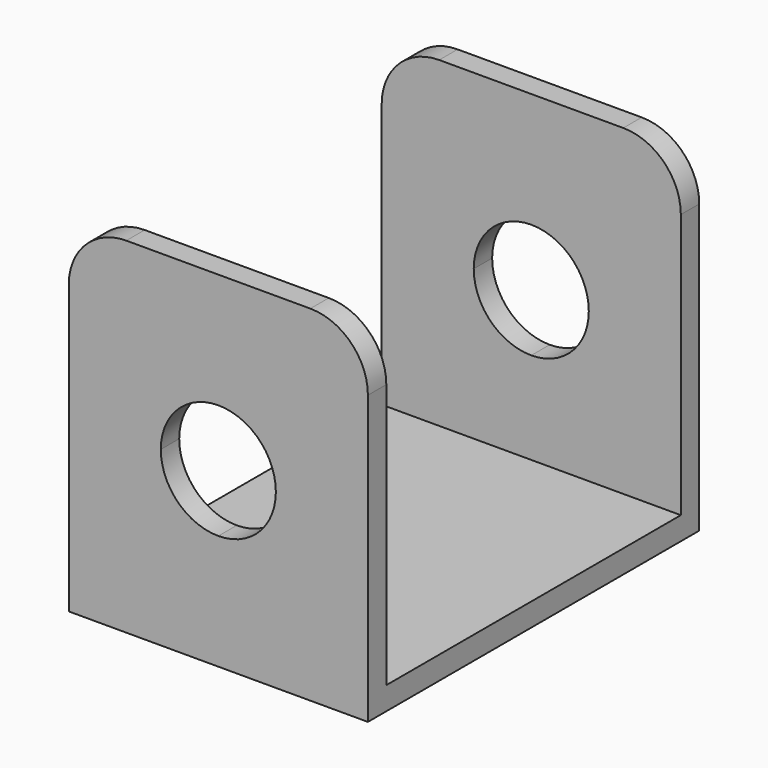
from build123d import *

# Parameters (mm, degrees)
F0_W     = 26
F0_H     = 2
F1_DEPTH = 30
F0_H_2   = 34
F2_DEPTH = 2
F4_DEPTH = 28
F5_R     = 5
F6_R     = 5
F9_DEPTH = 100


# Not quite as in the source:
# - a feature of the source that left no trace in its solid (it failed there, or was rolled back) is left out


with BuildPart() as f1:
    # F0 (on Top) → F1 (new body)
    with BuildSketch(Plane.XY):
        with Locations((0, 17)):
            Rectangle(F0_W, F0_H)
    extrude(amount=F1_DEPTH)

    # F0 (on Top) → F2 (join)
    with BuildSketch(Plane.XY):
        with Locations((0, -1)):
            Rectangle(F0_W, F0_H_2)
    extrude(amount=F2_DEPTH)

    # F3 (on face) → F4 (join)
    with BuildSketch(Plane.XY.offset(2)):
        Polygon((13, -16), (0, -16), (-13, -16), (-13, -18), (13, -18), align=None)
    extrude(amount=F4_DEPTH)

    # F5
    f5_edges = [f1.edges().sort_by_distance(p)[0] for p in [
        (-13, 17, 30),
        (-13, -17, 30),
    ]]
    fillet(f5_edges, radius=F5_R)

    # F6
    f6_edges = [f1.edges().sort_by_distance(p)[0] for p in [
        (13, 17, 30),
        (13, -17, 30),
    ]]
    fillet(f6_edges, radius=F6_R)

    # F8 (on face) → F9 (cut)
    with BuildSketch(Plane(origin=(0, 18, 0), x_dir=(-1, 0, 0), z_dir=(0, 1, 0))):
        with BuildLine():
            ThreePointArc((5, 15), (3.5355339059, 18.5355339059), (0, 20))
            Line((0, 20), (0, 10))
            ThreePointArc((0, 10), (3.5355339059, 11.4644660941), (5, 15))
        make_face()
        with BuildLine():
            Line((0, 10), (0, 20))
            ThreePointArc((0, 20), (-5, 15), (0, 10))
        make_face()
    extrude(amount=-F9_DEPTH, mode=Mode.SUBTRACT)


solid = f1.part
